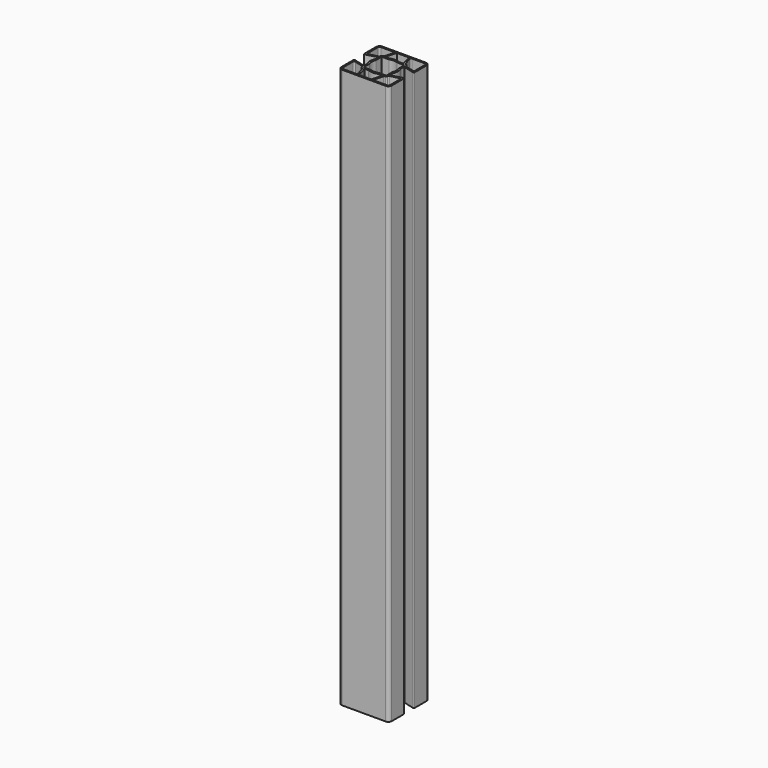
from build123d import *

# Parameters (mm, degrees)
F1_DEPTH = 1000


# Not quite as in the source:
# - ends of sketch curves that miss each other by under 0.0002 mm in the source are joined


with BuildPart() as f1:
    # F0 (on Top) → F1 (new body)
    with BuildSketch(Plane.XY):
        with BuildLine():
            ThreePointArc((23.0888885991, 8.8614578186), (23.022474706, 9.062799833), (23, 9.273618))
            Line((23, 9.273618), (23, 14.841657))
            ThreePointArc((23, 14.841657), (23.3912385359, 15.6350103133), (24.2588189596, 15.8075828492))
            Line((24.2588189596, 15.8075828492), (43.426476, 10.671624))
            ThreePointArc((43.426476, 10.671624), (44.5109517857, 10.8873403242), (45, 11.879032))
            Line((45, 11.879032), (45, 39))
            ThreePointArc((45, 39), (43.2426406871, 43.2426406871), (39, 45))
            Line((39, 45), (-39, 45))
            ThreePointArc((-39, 45), (-43.2426406871, 43.2426406871), (-45, 39))
            Line((-45, 39), (-45, 11.879032))
            ThreePointArc((-45, 11.879032), (-44.5109517857, 10.8873403242), (-43.4264761923, 10.6716247175))
            Line((-43.4264761923, 10.6716247175), (-24.258819, 15.807583))
            ThreePointArc((-24.258819, 15.807583), (-23.3912385359, 15.6350103133), (-23, 14.841657))
            Line((-23, 14.841657), (-23, 9.273618))
            ThreePointArc((-23, 9.273618), (-23.022474706, 9.062799833), (-23.0888885991, 8.8614578186))
            ThreePointArc((-23.0888885991, 8.8614578186), (-25, 0), (-23.0888887851, -8.8614579028))
            ThreePointArc((-23.0888887851, -8.8614579028), (-23.022474706, -9.062799833), (-23, -9.273618))
            Line((-23, -9.273618), (-23, -14.841657))
            ThreePointArc((-23, -14.841657), (-23.3912385359, -15.6350103133), (-24.2588189596, -15.8075828492))
            Line((-24.2588189596, -15.8075828492), (-43.426476, -10.671624))
            ThreePointArc((-43.426476, -10.671624), (-44.5109517857, -10.8873403242), (-45, -11.879032))
            Line((-45, -11.879032), (-45, -39))
            ThreePointArc((-45, -39), (-43.2426406871, -43.2426406871), (-39, -45))
            Line((-39, -45), (39, -45))
            ThreePointArc((39, -45), (43.2426406871, -43.2426406871), (45, -39))
            Line((45, -39), (45, -11.879032))
            ThreePointArc((45, -11.879032), (44.5109517857, -10.8873403242), (43.4264761923, -10.6716247175))
            Line((43.4264761923, -10.6716247175), (24.258819, -15.807583))
            ThreePointArc((24.258819, -15.807583), (23.3912385359, -15.6350103133), (23, -14.841657))
            Line((23, -14.841657), (23, -9.273618))
            ThreePointArc((23, -9.273618), (23.022474706, -9.062799833), (23.0888885991, -8.8614578186))
            ThreePointArc((23.0888885991, -8.8614578186), (25, 0), (23.0888885991, 8.8614578186))
        make_face()
        with BuildLine():
            Line((-14.841657, -23), (-9.273618, -23))
            ThreePointArc((-9.273618, -23), (-9.062799833, -23.022474706), (-8.8614578186, -23.0888885991))
            ThreePointArc((-8.8614578186, -23.0888885991), (0, -25), (8.8614579028, -23.0888887851))
            ThreePointArc((8.8614579028, -23.0888887851), (9.062799833, -23.022474706), (9.273618, -23))
            Line((9.273618, -23), (14.841657, -23))
            ThreePointArc((14.841657, -23), (15.6350103133, -23.3912385359), (15.8075828492, -24.2588189596))
            Line((15.8075828492, -24.2588189596), (10.98686, -42.25))
            Line((10.98686, -42.25), (-10.98686, -42.25))
            Line((-10.98686, -42.25), (-15.807583, -24.258819))
            ThreePointArc((-15.807583, -24.258819), (-15.6350103133, -23.3912385359), (-14.841657, -23))
        make_face(mode=Mode.SUBTRACT)
        with BuildLine():
            Line((-39.732362, -14.508469), (-24.482362, -18.594694))
            ThreePointArc((-24.482362, -18.594694), (-23.4132933733, -19.3090230718), (-23, -20.526546))
            Line((-23, -20.526546), (-23, -21))
            ThreePointArc((-23, -21), (-22.4142135624, -22.4142135624), (-21, -23))
            Line((-21, -23), (-20.526546, -23))
            ThreePointArc((-20.526546, -23), (-19.3090230718, -23.4132933733), (-18.5946943016, -24.4823620808))
            Line((-18.5946943016, -24.4823620808), (-14.508469, -39.732362))
            ThreePointArc((-14.508469, -39.732362), (-14.8536143733, -41.4675229282), (-16.440321, -42.25))
            Line((-16.440321, -42.25), (-39, -42.25))
            ThreePointArc((-39, -42.25), (-41.2980970389, -41.2980970389), (-42.25, -39))
            Line((-42.25, -39), (-42.25, -16.440321))
            ThreePointArc((-42.25, -16.440321), (-41.4675229282, -14.8536143733), (-39.732362, -14.508469))
        make_face(mode=Mode.SUBTRACT)
        with BuildLine():
            Line((14.508469, -39.732362), (18.594694, -24.482362))
            ThreePointArc((18.594694, -24.482362), (19.3090230718, -23.4132933733), (20.526546, -23))
            Line((20.526546, -23), (21, -23))
            ThreePointArc((21, -23), (22.4142135624, -22.4142135624), (23, -21))
            Line((23, -21), (23, -20.526546))
            ThreePointArc((23, -20.526546), (23.4132933733, -19.3090230718), (24.4823620808, -18.5946943016))
            Line((24.4823620808, -18.5946943016), (39.732362, -14.508469))
            ThreePointArc((39.732362, -14.508469), (41.4675229282, -14.8536143733), (42.25, -16.440321))
            Line((42.25, -16.440321), (42.25, -39))
            ThreePointArc((42.25, -39), (41.2980970389, -41.2980970389), (39, -42.25))
            Line((39, -42.25), (16.440321, -42.25))
            ThreePointArc((16.440321, -42.25), (14.8536143733, -41.4675229282), (14.508469, -39.732362))
        make_face(mode=Mode.SUBTRACT)
        with BuildLine():
            Line((-7.3951, -20.25), (-19.25, -20.25))
            ThreePointArc((-19.25, -20.25), (-19.9571067812, -19.9571067812), (-20.25, -19.25))
            Line((-20.25, -19.25), (-20.25, -7.3951))
            ThreePointArc((-20.25, -7.3951), (-20.2639867072, -7.2284333074), (-20.3055555728, -7.0664288513))
            ThreePointArc((-20.3055554887, -7.066428822), (-21.5, 0), (-20.3055554887, 7.066428822))
            ThreePointArc((-20.3055555728, 7.0664288513), (-20.2639867072, 7.2284333074), (-20.25, 7.3951))
            Line((-20.25, 7.3951), (-20.25, 19.25))
            ThreePointArc((-20.25, 19.25), (-19.9571067812, 19.9571067812), (-19.25, 20.25))
            Line((-19.25, 20.25), (-7.3951, 20.25))
            ThreePointArc((-7.3951, 20.25), (-7.2284333074, 20.2639867072), (-7.0664288513, 20.3055555728))
            ThreePointArc((-7.066428822, 20.3055554887), (0, 21.5), (7.066428822, 20.3055554887))
            ThreePointArc((7.0664288513, 20.3055555728), (7.2284333074, 20.2639867072), (7.3951, 20.25))
            Line((7.3951, 20.25), (19.25, 20.25))
            ThreePointArc((19.25, 20.25), (19.9571067812, 19.9571067812), (20.25, 19.25))
            Line((20.25, 19.25), (20.25, 7.3951))
            ThreePointArc((20.25, 7.3951), (20.2639867072, 7.2284333074), (20.3055555728, 7.0664288513))
            ThreePointArc((20.3055554887, 7.066428822), (21.5, 0), (20.3055554887, -7.066428822))
            ThreePointArc((20.3055555728, -7.0664288513), (20.2639867072, -7.2284333074), (20.25, -7.3951))
            Line((20.25, -7.3951), (20.25, -19.25))
            ThreePointArc((20.25, -19.25), (19.9571067812, -19.9571067812), (19.25, -20.25))
            Line((19.25, -20.25), (7.3951, -20.25))
            ThreePointArc((7.3951, -20.25), (7.2284333074, -20.2639867072), (7.0664288513, -20.3055555728))
            ThreePointArc((7.066428822, -20.3055554887), (0, -21.5), (-7.066428822, -20.3055554887))
            ThreePointArc((-7.0664288513, -20.3055555728), (-7.2284333074, -20.2639867072), (-7.3951, -20.25))
        make_face(mode=Mode.SUBTRACT)
        with BuildLine():
            Line((-14.508469, 39.732362), (-18.594694, 24.482362))
            ThreePointArc((-18.594694, 24.482362), (-19.3090230718, 23.4132933733), (-20.526546, 23))
            Line((-20.526546, 23), (-21, 23))
            ThreePointArc((-21, 23), (-22.4142135624, 22.4142135624), (-23, 21))
            Line((-23, 21), (-23, 20.526546))
            ThreePointArc((-23, 20.526546), (-23.4132933733, 19.3090230718), (-24.4823620808, 18.5946943016))
            Line((-24.4823620808, 18.5946943016), (-39.732362, 14.508469))
            ThreePointArc((-39.732362, 14.508469), (-41.4675229282, 14.8536143733), (-42.25, 16.440321))
            Line((-42.25, 16.440321), (-42.25, 39))
            ThreePointArc((-42.25, 39), (-41.2980970389, 41.2980970389), (-39, 42.25))
            Line((-39, 42.25), (-16.440321, 42.25))
            ThreePointArc((-16.440321, 42.25), (-14.8536143733, 41.4675229282), (-14.508469, 39.732362))
        make_face(mode=Mode.SUBTRACT)
        with BuildLine():
            Line((-15.807583, 24.258819), (-10.98686, 42.25))
            Line((-10.98686, 42.25), (10.98686, 42.25))
            Line((10.98686, 42.25), (15.807583, 24.258819))
            ThreePointArc((15.807583, 24.258819), (15.6350103133, 23.3912385359), (14.841657, 23))
            Line((14.841657, 23), (9.273618, 23))
            ThreePointArc((9.273618, 23), (9.062799833, 23.022474706), (8.8614578186, 23.0888885991))
            ThreePointArc((8.8614578186, 23.0888885991), (0, 25), (-8.8614579028, 23.0888887851))
            ThreePointArc((-8.8614579028, 23.0888887851), (-9.062799833, 23.022474706), (-9.273618, 23))
            Line((-9.273618, 23), (-14.841657, 23))
            ThreePointArc((-14.841657, 23), (-15.6350103133, 23.3912385359), (-15.807583, 24.258819))
        make_face(mode=Mode.SUBTRACT)
        with BuildLine():
            Line((39.732362, 14.508469), (24.482362, 18.594694))
            ThreePointArc((24.482362, 18.594694), (23.4132933733, 19.3090230718), (23, 20.526546))
            Line((23, 20.526546), (23, 21))
            ThreePointArc((23, 21), (22.4142135624, 22.4142135624), (21, 23))
            Line((21, 23), (20.526546, 23))
            ThreePointArc((20.526546, 23), (19.3090230718, 23.4132933733), (18.5946943016, 24.4823620808))
            Line((18.5946943016, 24.4823620808), (14.508469, 39.732362))
            ThreePointArc((14.508469, 39.732362), (14.8536143733, 41.4675229282), (16.440321, 42.25))
            Line((16.440321, 42.25), (39, 42.25))
            ThreePointArc((39, 42.25), (41.2980970389, 41.2980970389), (42.25, 39))
            Line((42.25, 39), (42.25, 16.440321))
            ThreePointArc((42.25, 16.440321), (41.4675229282, 14.8536143733), (39.732362, 14.508469))
        make_face(mode=Mode.SUBTRACT)
    extrude(amount=F1_DEPTH)


solid = f1.part
